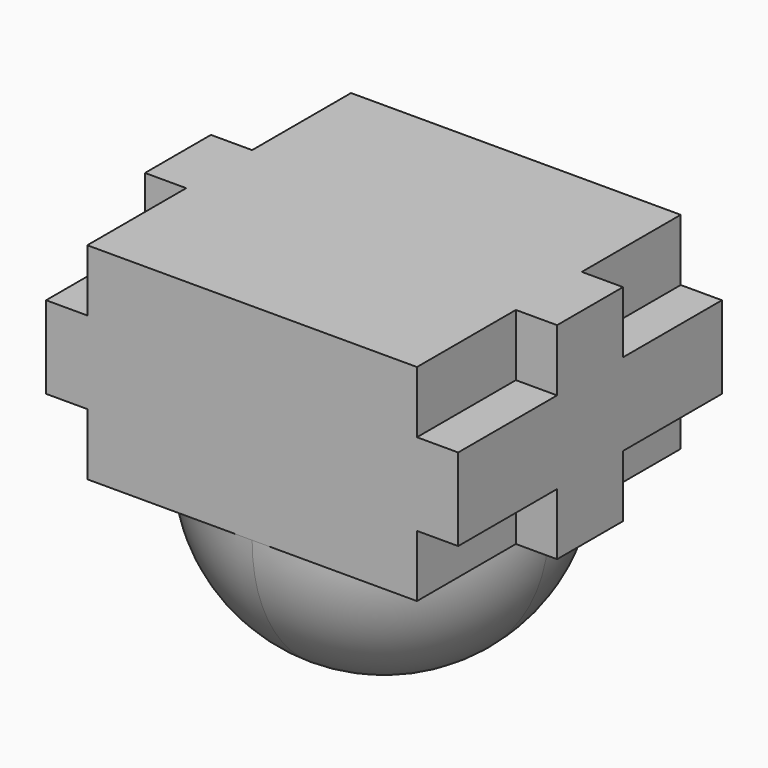
from build123d import *

# Parameters (mm, degrees)
F0_W     = 40
F0_H     = 40
F1_DEPTH = 40
F2_R     = 19.99999
F3_W     = 40
F3_H     = 40
F4_DEPTH = 25
F6_DEPTH = 25
F7_DEPTH = 50


# Not quite as in the source:
# - a fillet or chamfer is up to 0.001 mm smaller than in the source, because OpenCascade refuses the exact size


with BuildPart() as f1:
    # F0 (on Front) → F1 (new body)
    with BuildSketch(Plane.XZ):
        Rectangle(F0_W, F0_H)
    extrude(amount=F1_DEPTH)

    # F2 (radius 20 in the source; OpenCascade refuses exactly that, so slightly less here)
    f2_edges = [f1.edges().sort_by_distance(p)[0] for p in [
        (20, -20, 20),
        (-20, -20, 20),
        (0, 0, 20),
        (0, -40, 20),
        (0, -40, -20),
        (20, -40, 0),
        (-20, -40, 0),
        (20, -20, -20),
        (20, 0, 0),
        (0, 0, -20),
        (-20, 0, 0),
        (-20, -20, -20),
    ]]
    fillet(f2_edges, radius=F2_R)

    # F3 (on Top) → F4 (join)
    with BuildSketch(Plane.XY):
        with Locations((0, -20)):
            Rectangle(F3_W, F3_H)
    extrude(amount=F4_DEPTH)

    # F5 (on Right) → F6 (join)
    with BuildSketch(Plane.YZ):
        Polygon((-25, 0), (-20, 0), (-15, 0), (-15, 7.5), (0, 7.5), (0, 17.5), (-15, 17.5), (-15, 25), (-25, 25), (-25, 17.5), (-40, 17.5), (-40, 7.5), (-25, 7.5), align=None)
    extrude(amount=F6_DEPTH)

    # F7 (add): a face of the model
    f7_faces = [f1.faces().sort_by_distance(p)[0] for p in [
        (25, -20, 12.5),
    ]]
    extrude(f7_faces, amount=-F7_DEPTH)


solid = f1.part
